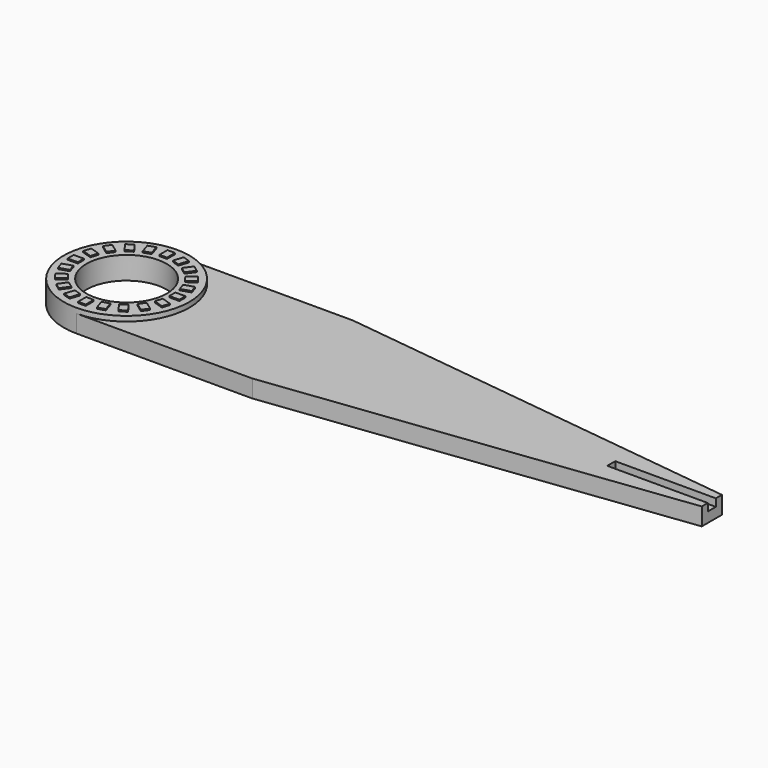
from build123d import *

# Parameters (mm, degrees)
F0_R         = 8
F1_DEPTH     = 3.5
F2_R         = 12.5
F2_R_2       = 8
F3_DEPTH     = 1
F4_W         = 1.5
F4_H         = 2
F4_W_2       = 2
F4_H_2       = 1.5
F5_DEPTH     = 0.25
F6_W         = 20
F6_H         = 2
F7_DEPTH     = 1.5
F9_TEXT_SIZE = 16.6499423942
F10_DEPTH    = 1.5


# Not quite as in the source:
# - Text() gives the source's letters only with a copy of the font that has no kerning and outlines rounded to 1/6400 em; it was checked with that copy


with BuildPart() as f1:
    # F0 (on Top) → F1 (new body)
    with BuildSketch(Plane.XY):
        with BuildLine():
            Line((35, 12.5), (0, 12.5))
            ThreePointArc((0, 12.5), (-12.5, 0), (0, -12.5))
            Line((0, -12.5), (35, -12.5))
            Line((35, -12.5), (116.3887844346, -2.5067138408))
            Line((116.3887844346, -2.5067138408), (116.3887844346, 2.5067138408))
            Line((116.3887844346, 2.5067138408), (35, 12.5))
        make_face()
        Circle(F0_R, mode=Mode.SUBTRACT)
    extrude(amount=F1_DEPTH)

    # F2 (on face) → F3 (join)
    with BuildSketch(Plane.XY.offset(3.5)):
        Circle(F2_R)
        Circle(F2_R_2, mode=Mode.SUBTRACT)
    extrude(amount=F3_DEPTH)

    # F4 (on face) → F5 (join)
    with BuildSketch(Plane.XY.offset(4.5)):
        with Locations((0, 10.1045304909)):
            Rectangle(F4_W, F4_H)
        Polygon((-2.1001622603, 8.890685797), (-2.718196249, 10.7927988296), (-4.1447810235, 10.329273338), (-3.5267470347, 8.4271603054), align=None)
        Polygon((-4.7447460058, 7.8065588322), (-5.9203165104, 9.4245928209), (-7.133842002, 8.5429149425), (-5.9582714974, 6.9248809538), align=None)
        Polygon((-6.9248809538, 5.9582714974), (-8.5429149425, 7.133842002), (-9.4245928209, 5.9203165104), (-7.8065588322, 4.7447460058), align=None)
        Polygon((-8.4271603054, 3.5267470347), (-10.329273338, 4.1447810235), (-10.7927988296, 2.718196249), (-8.890685797, 2.1001622603), align=None)
        with Locations((-10.1045304909, 0)):
            Rectangle(F4_W_2, F4_H_2)
        Polygon((-8.890685797, -2.1001622603), (-10.7927988296, -2.718196249), (-10.329273338, -4.1447810235), (-8.4271603054, -3.5267470347), align=None)
        Polygon((-7.8065588322, -4.7447460058), (-9.4245928209, -5.9203165104), (-8.5429149425, -7.133842002), (-6.9248809538, -5.9582714974), align=None)
        Polygon((-5.9582714974, -6.9248809538), (-7.133842002, -8.5429149425), (-5.9203165104, -9.4245928209), (-4.7447460058, -7.8065588322), align=None)
        Polygon((-3.5267470347, -8.4271603054), (-4.1447810235, -10.329273338), (-2.718196249, -10.7927988296), (-2.1001622603, -8.890685797), align=None)
        with Locations((0, -10.1045304909)):
            Rectangle(F4_W, F4_H)
        Polygon((2.1001622603, -8.890685797), (2.718196249, -10.7927988296), (4.1447810235, -10.329273338), (3.5267470347, -8.4271603054), align=None)
        Polygon((4.7447460058, -7.8065588322), (5.9203165104, -9.4245928209), (7.133842002, -8.5429149425), (5.9582714974, -6.9248809538), align=None)
        Polygon((6.9248809538, -5.9582714974), (8.5429149425, -7.133842002), (9.4245928209, -5.9203165104), (7.8065588322, -4.7447460058), align=None)
        Polygon((8.4271603054, -3.5267470347), (10.329273338, -4.1447810235), (10.7927988296, -2.718196249), (8.890685797, -2.1001622603), align=None)
        with Locations((10.1045304909, 0)):
            Rectangle(F4_W_2, F4_H_2)
        Polygon((8.890685797, 2.1001622603), (10.7927988296, 2.718196249), (10.329273338, 4.1447810235), (8.4271603054, 3.5267470347), align=None)
        Polygon((7.8065588322, 4.7447460058), (9.4245928209, 5.9203165104), (8.5429149425, 7.133842002), (6.9248809538, 5.9582714974), align=None)
        Polygon((5.9582714974, 6.9248809538), (7.133842002, 8.5429149425), (5.9203165104, 9.4245928209), (4.7447460058, 7.8065588322), align=None)
        Polygon((3.5267470347, 8.4271603054), (4.1447810235, 10.329273338), (2.718196249, 10.7927988296), (2.1001622603, 8.890685797), align=None)
    extrude(amount=F5_DEPTH)

    # F6 (on face) → F7 (cut)
    with BuildSketch(Plane.XY.offset(3.5)):
        with Locations((106.3887844346, -0.0067138408)):
            Rectangle(F6_W, F6_H)
    extrude(amount=-F7_DEPTH, mode=Mode.SUBTRACT)

    # F9 (on face) → F10 (cut)
    with BuildSketch(Plane(origin=(0, 0, 0), x_dir=(1, 0, 0), z_dir=(0, 0, -1))):
        with Locations((10, -5.9939792619)):
            Text('Adrienne', F9_TEXT_SIZE, font='Open Sans', text_align=(TextAlign.LEFT, TextAlign.BOTTOM))
    extrude(amount=-F10_DEPTH, mode=Mode.SUBTRACT)


solid = f1.part
